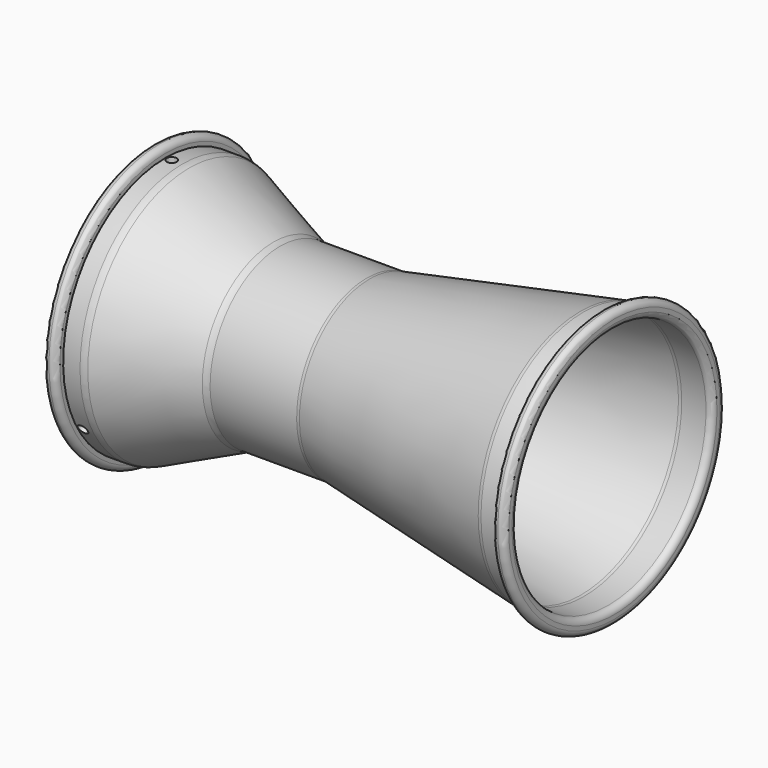
from build123d import *

# Parameters (mm, degrees)
F2_R     = 8
F3_R     = 2.99999
F4_R     = 4
F4_R_2   = 20
F5_DEPTH = 157.0010001
F6_R     = 2.5
F7_DEPTH = 68.101
F8_COUNT = 3


# Not quite as in the source:
# - a fillet or chamfer is up to 0.001 mm smaller than in the source, because OpenCascade refuses the exact size


with BuildPart() as f1:
    # F0 (on Front) → F1 (revolve)
    with BuildSketch(Plane.XZ):
        Polygon((6, 68.1), (0, 68.1), (0, 60.1), (15.3586869108, 60.1), (60, 40.1), (70, 40.1), (70, 0), (76, 0), (76, 40.1), (106, 40.1), (211.2824225013, 60.1), (227, 60.1), (227, 68.1), (221, 68.1), (221, 63.1), (211, 63.1), (105.7175774987, 43.1), (60.6413130892, 43.1), (16, 63.1), (6, 63.1), align=None)
    revolve(axis=Axis((99.3098750351, 0, 0), (1, 0, 0)))

    # F2
    f2_edges = [f1.edges().sort_by_distance(p)[0] for p in [
        (16, 0, -63.1),
        (211, 0, -63.1),
        (105.717577, 0, -43.1),
        (60.641313, 0, -43.1),
        (15.358687, 0, -60.1),
        (211.282423, 0, -60.1),
    ]]
    fillet(f2_edges, radius=F2_R)

    # F3 (radius 3 in the source; OpenCascade refuses exactly that, so slightly less here)
    f3_edges = [f1.edges().sort_by_distance(p)[0] for p in [
        (0, 0, -68.1),
        (6, 0, -68.1),
        (221, 0, -68.1),
        (227, 0, -68.1),
        (0, 0, -60.1),
        (60, 0, -40.1),
        (70, 0, -40.1),
        (227, 0, -60.1),
        (76, 0, -40.1),
        (106, 0, -40.1),
    ]]
    fillet(f3_edges, radius=F3_R)

    # F4 (on face) → F5 (cut, through all)
    with BuildSketch(Plane(origin=(70, 0, 0), x_dir=(0, -1, 0), z_dir=(-1, 0, 0))):
        with Locations((0, 30)):
            Circle(F4_R)
        with Locations((30, 0)):
            Circle(F4_R)
        with Locations((0, -30)):
            Circle(F4_R)
        with Locations((-30, 0)):
            Circle(F4_R)
        Circle(F4_R_2)
    extrude(amount=-F5_DEPTH, mode=Mode.SUBTRACT)

    # F6 (on Top) → F7 (cut, through all)
    with BuildSketch(Plane.XY):
        with Locations((9, 0)):
            Circle(F6_R)
    f7 = extrude(amount=F7_DEPTH, mode=Mode.SUBTRACT)

    # F8: F7 ×3 about axis
    f8_axis = Axis((106, 0, 0), (1, 0, 0))
    for i in range(1, F8_COUNT):
        add(f7.rotate(f8_axis, i * 360 / F8_COUNT), mode=Mode.SUBTRACT)


solid = f1.part
